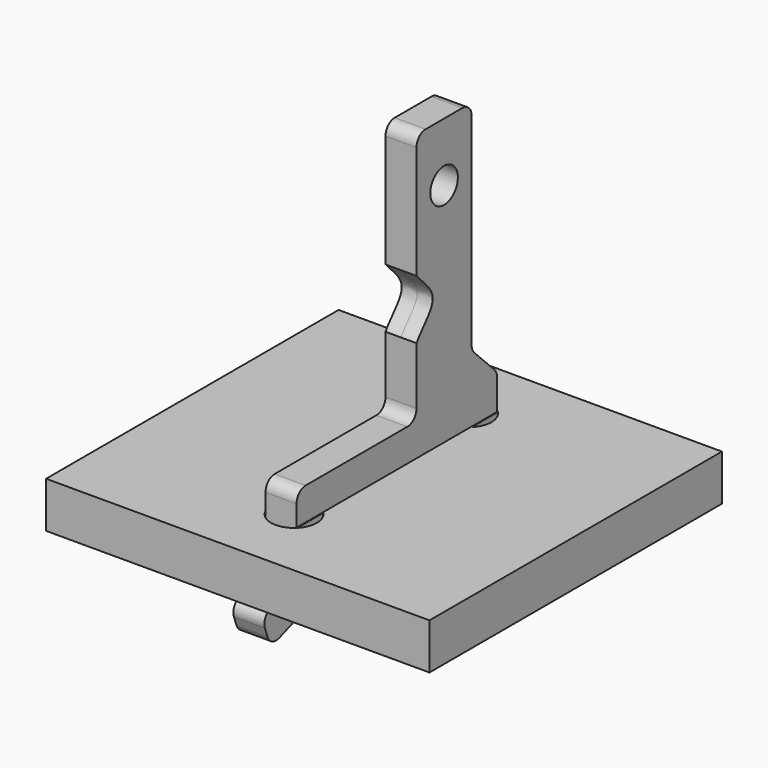
from build123d import *

# Parameters (mm, degrees)
F1_W        = 33.3865592256
F1_H        = 31.8326419219
F2_DEPTH    = 4
F1_W_2      = 2.8284271247
F1_H_2      = 2.8284271247
F3_DEPTH    = 4
F4_R        = 1.5
F5_DEPTH    = 1.35
F6_T4_DEPTH = 2.7
F7_R        = 3.8
F8_R        = 1


# Not quite as in the source:
# - a fillet or chamfer that OpenCascade refuses, or shapes differently, is made with other operations: its cross-section is extruded or revolved along the edge and cut away or added


with BuildPart() as f2:
    # F1 (on Top) → F2 (new body)
    with BuildSketch(Plane.XY):
        with Locations((0.2483981661, 9.4852247275)):
            Rectangle(F1_W, F1_H)
        with BuildLine():
            ThreePointArc((1.4142135624, 1.4142135624), (1.847759065, 0.7653668647), (2, 0))
            ThreePointArc((2, 0), (1.847759065, -0.7653668647), (1.4142135624, -1.4142135624))
            ThreePointArc((1.4142135624, -1.4142135624), (0, -2), (-1.4142135624, -1.4142135624))
            ThreePointArc((-1.4142135624, -1.4142135624), (-2, 0), (-1.4142135624, 1.4142135624))
            ThreePointArc((-1.4142135624, 1.4142135624), (0, 2), (1.4142135624, 1.4142135624))
        make_face(mode=Mode.SUBTRACT)
        with BuildLine():
            ThreePointArc((1.4142135624, 20.4142135624), (1.847759065, 19.7653668647), (2, 19))
            ThreePointArc((2, 19), (1.847759065, 18.2346331353), (1.4142135624, 17.5857864376))
            ThreePointArc((1.4142135624, 17.5857864376), (0, 17), (-1.4142135624, 17.5857864376))
            ThreePointArc((-1.4142135624, 17.5857864376), (-2, 19), (-1.4142135624, 20.4142135624))
            ThreePointArc((-1.4142135624, 20.4142135624), (0, 21), (1.4142135624, 20.4142135624))
        make_face(mode=Mode.SUBTRACT)
    extrude(amount=F2_DEPTH)


with BuildPart() as f3:
    # F1 (on Top) → F3 (new body)
    with BuildSketch(Plane.XY):
        Rectangle(F1_W_2, F1_H_2)
    extrude(amount=F3_DEPTH)


with BuildPart() as f3b:
    # F1 (on Top) → F3, piece 2 (new body)
    with BuildSketch(Plane.XY):
        with Locations((0, 19)):
            Rectangle(F1_W_2, F1_H_2)
    extrude(amount=F3_DEPTH)


with BuildPart() as f5:
    # F4 (on Right) → F5 (new body, symmetric)
    with BuildSketch(Plane.YZ):
        with BuildLine():
            Line((-1.4142135624, 6.828), (-1.4142135624, 4))
            Line((-1.4142135624, 4), (-1.4142135624, 0))
            Line((-1.4142135624, 0), (-5.1972519021, -1.3769133508))
            Line((-5.1972519021, -1.3769133508), (-4.2300189368, -4.0343640823))
            Line((-4.2300189368, -4.0343640823), (1.4142135624, -1.9800314574))
            Line((1.4142135624, -1.9800314574), (1.4142135624, 0))
            Line((1.4142135624, 0), (1.4142135624, 4))
            Line((1.4142135624, 4), (17.5857864376, 4))
            Line((17.5857864376, 4), (17.5857864376, 0))
            Line((17.5857864376, 0), (17.5857864376, -2))
            Line((17.5857864376, -2), (20.4142135624, -2))
            Line((20.4142135624, -2), (20.4142135624, 0))
            Line((20.4142135624, 0), (20.4142135624, 4))
            Line((20.4142135624, 4), (20.4142135624, 6.828))
            Line((20.4142135624, 6.828), (17.646729894, 6.828))
            Line((17.646729894, 6.828), (17.646729894, 28.828))
            Line((17.646729894, 28.828), (11.646729894, 28.828))
            Line((11.646729894, 28.828), (11.646729894, 17.9849732667))
            add(Edge.make_bspline(
                [(11.646729894, 12.828), (12.1738818895, 13.7014529164), (14.6496330846, 15.5152462823), (12.174934911, 17.339967343), (11.646729894, 17.9849732667)],
                knots=[0, 0, 0, 0, 0.5096847631, 1, 1, 1, 1], degree=3))
            Line((11.646729894, 12.828), (11.646729894, 6.828))
            Line((11.646729894, 6.828), (-1.4142135624, 6.828))
        make_face()
        with Locations((14.646729894, 23.7077325583)):
            Circle(F4_R, mode=Mode.SUBTRACT)
    extrude(amount=F5_DEPTH, both=True)

    # F6: chamfer of 3 on 1 edges, made by hand


with BuildPart() as f6_tool2:
    # F6_s3 → F6_t4 (new body)
    with BuildSketch(Plane.YZ.offset(-1.35)):
        Polygon((17.646729894, 9.828), (20.646729894, 6.828), (17.646729894, 6.828), align=None)
    extrude(amount=F6_T4_DEPTH)

    split(bisect_by=Plane.XZ.offset(-20.4142135624), keep=Keep.TOP)


with BuildPart() as f5_1:
    add(f5.part)

    # F6_t1: union F6_tool2
    add(f6_tool2.part)

    # F7
    f7_edges = [f5_1.edges().sort_by_distance(p)[0] for p in [
        (0, 1.414214, -1.980031),
    ]]
    fillet(f7_edges, radius=F7_R)

    # F8
    f8_edges = [f5_1.edges().sort_by_distance(p)[0] for p in [
        (0, -5.197252, -1.376913),
        (0, -4.230019, -4.034364),
        (0, -1.414214, 6.828),
        (0, 11.64673, 6.828),
        (0, 11.64673, 28.828),
        (0, 17.64673, 28.828),
        (0, 17.585786, -2),
        (0, 20.414214, -2),
        (0, 20.414214, 7.060516),
        (0, 17.64673, 9.828),
    ]]
    fillet(f8_edges, radius=F8_R)


solid = Compound([f2.part, f3.part, f3b.part, f5_1.part])
